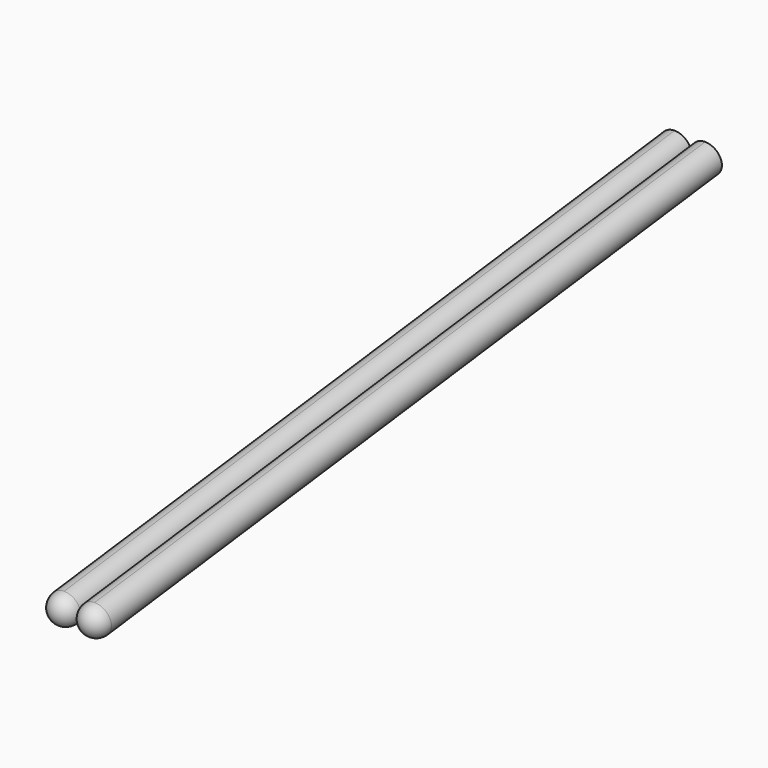
from build123d import *

# Parameters (mm, degrees)
F14_DEPTH      = 0.508
F14_DEPTH_BACK = 0.508
F15_T1_DEPTH   = 12.0876033166
F16_T1_DEPTH   = 11.7701033166


# Not quite as in the source:
# - a fillet or chamfer that OpenCascade refuses, or shapes differently, is made with other operations: its cross-section is extruded or revolved along the edge and cut away or added


with BuildPart() as f7:
    # F5 (on offset) → F7 (revolve)
    with BuildSketch(Plane.YZ.offset(0.508)):
        Polygon((-25.4, 0), (0, 3.175), (-0.0630096452, 3.6790771614), (-25.4630096452, 0.5040771614), align=None)
    revolve(axis=Axis((0.508, -12.7, 1.5875), (0, -0.9922778767, -0.1240347346)))



with BuildPart() as f8:
    # F6 (on offset) → F8 (revolve)
    with BuildSketch(Plane.YZ.offset(-0.508)):
        Polygon((-25.4, 0), (0, 3.175), (-0.0630096452, 3.6790771614), (-25.4630096452, 0.5040771614), align=None)
    revolve(axis=Axis((-0.508, -12.7, 1.5875), (0, -0.9922778767, -0.1240347346)))

    # F9 (on offset) → F11 (revolve)
    with BuildSketch(Plane.XZ.offset(25.4)):
        with BuildLine():
            ThreePointArc((-1.016, 0), (-0.508, -0.508), (0, 0))
            Line((0, 0), (-1.016, 0))
        make_face()
    revolve(axis=Axis((-0.508, -25.4, 0), (-1, 0, 0)))


with BuildPart() as f7_1:
    add(f7.part)

    add(f8.part)  # F12 merges F8
    # F10 (on offset) → F12 (revolve)
    with BuildSketch(Plane.XZ.offset(25.4)):
        with BuildLine():
            ThreePointArc((0, 0), (0.508, -0.508), (1.016, 0))
            Line((1.016, 0), (0, 0))
        make_face()
    revolve(axis=Axis((0.508, -25.4, 0), (1, 0, 0)))


with BuildPart() as f14:
    # F13 (on Right) → F14 (new body, two sides)
    with BuildSketch(Plane.YZ) as f14_sk:
        Polygon((-19.05, 0.281796633), (-19.05, 0.79375), (-25.4, 0), (-25.3369903548, -0.5040771614), align=None)
    extrude(amount=F14_DEPTH)
    extrude(f14_sk.sketch, amount=-F14_DEPTH_BACK)

    # F15: fillet of radius 5.08 on 1 edges, made by hand

    # F15_s2 → F15_t1 (cut)
    with BuildSketch(Plane.YZ.offset(-6.0438016583)):
        with BuildLine():
            ThreePointArc((-23.1397689487, -0.2294244856), (-24.2828741459, -0.2426831475), (-25.4, 0))
            Line((-25.4, 0), (-25.3369903548, -0.5040771614))
            Line((-25.3369903548, -0.5040771614), (-23.1397689487, -0.2294244856))
        make_face()
    extrude(amount=F15_T1_DEPTH, mode=Mode.SUBTRACT)

    # F16: fillet of radius 5.08 on 1 edges, made by hand

    # F16_s2 → F16_t1 (cut)
    with BuildSketch(Plane.YZ.offset(-5.8850516583)):
        with BuildLine():
            ThreePointArc((-19.05, 0.79375), (-20.0730153607, 0.2835492006), (-21.184211761, 0.0150201629))
            Line((-21.184211761, 0.0150201629), (-19.05, 0.281796633))
            Line((-19.05, 0.281796633), (-19.05, 0.79375))
        make_face()
    extrude(amount=F16_T1_DEPTH, mode=Mode.SUBTRACT)


solid = Compound([f7_1.part, f14.part])
